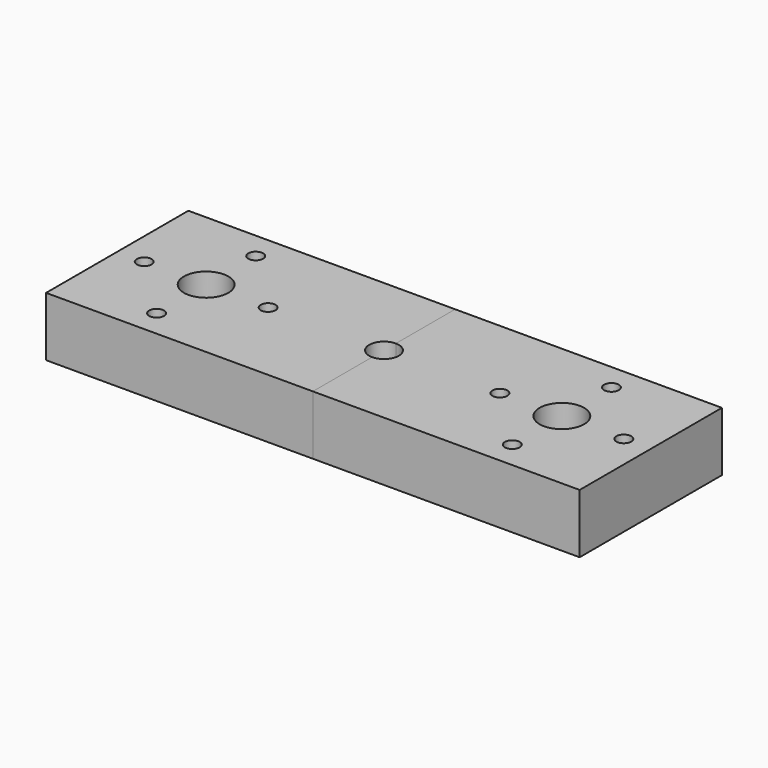
from build123d import *
from build123d import SkipClean  # not in build123d's __all__

# Parameters (mm, degrees)
F0_R     = 3.175
F0_R_2   = 9.525
F1_DEPTH = 25.4


# Not quite as in the source:
# - a pattern or mirror of a feature is missing from the dataset's text; its kind, count and spacing are read off the source's solid


with BuildPart() as f1:
    # F0 (on Top) → F1 (new body)
    with BuildSketch(Plane.XY):
        with BuildLine():
            Line((0, 38.1), (-114.3, 38.1))
            Line((-114.3, 38.1), (-114.3, -38.1))
            Line((-114.3, -38.1), (0, -38.1))
            Line((0, -38.1), (0, -6.35))
            ThreePointArc((0, -6.35), (-6.35, 0), (0, 6.35))
            Line((0, 6.35), (0, 38.1))
        make_face()
        with Locations((-76.2, -26.543)):
            Circle(F0_R, mode=Mode.SUBTRACT)
        with Locations((-102.743, 0)):
            Circle(F0_R, mode=Mode.SUBTRACT)
        with Locations((-76.2, 0)):
            Circle(F0_R_2, mode=Mode.SUBTRACT)
        with Locations((-76.2, 26.543)):
            Circle(F0_R, mode=Mode.SUBTRACT)
        with Locations((-49.657, 0)):
            Circle(F0_R, mode=Mode.SUBTRACT)
    extrude(amount=F1_DEPTH)

    # F1_copies: F1 across plane


with BuildPart() as f1_1:
    add(f1.part, clean=False)
    with SkipClean():  # cleaning this boolean's faces spoils the solid; the shape is the same uncleaned
        add(f1.part.mirror(Plane(origin=(0, 0, 0), x_dir=(0, 0, 1), z_dir=(1, 0, 0))), clean=False)


solid = f1_1.part
